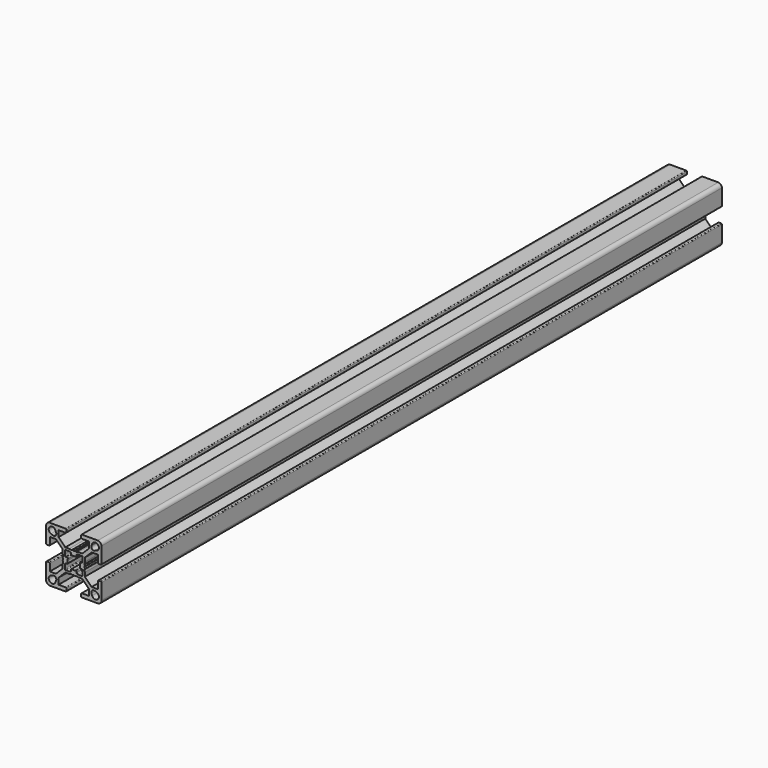
from build123d import *

# Parameters (mm, degrees)
F1_DEPTH = 420


# Not quite as in the source:
# - ends of sketch curves that miss each other by under 0.0002 mm in the source are joined


with BuildPart() as f1:
    # F0 (on Front) → F1 (new body)
    with BuildSketch(Plane.XZ):
        with BuildLine():
            ThreePointArc((21.683673, 22.959406), (21.8008302875, 23.2422487125), (22.083673, 23.359406))
            Line((22.083673, 23.359406), (23.829607, 23.359406))
            ThreePointArc((23.829607, 23.359406), (23.8679454853, 23.3575644616), (23.9059309617, 23.3520568027))
            Line((23.9059309617, 23.3520568027), (24.659993, 23.205482))
            ThreePointArc((24.659993, 23.205482), (24.8923196389, 23.067262524), (24.98367, 22.812831))
            Line((24.98367, 22.812831), (24.98367, 22.196712))
            ThreePointArc((24.98367, 22.196712), (25.1452540389, 21.8755300741), (25.4994591475, 21.8138375123))
            ThreePointArc((25.4994591475, 21.8138375123), (25.9862111121, 21.9228171635), (26.48367, 21.959406))
            Line((26.48367, 21.959406), (26.48367, 24.259406))
            Line((26.48367, 24.259406), (26.080079, 24.492418))
            ThreePointArc((26.080079, 24.492418), (25.830079, 24.559406), (25.5800791291, 24.4924187764))
            Line((25.5800791291, 24.4924187764), (25.264783, 24.310382))
            Line((25.264783, 24.310382), (23.98367, 24.559406))
            Line((23.98367, 24.559406), (21.897875, 24.559406))
            Line((21.897875, 24.559406), (18.23367, 28.223612))
            Line((18.23367, 28.223612), (18.23367, 31.559402))
            Line((18.23367, 31.559402), (22.083673, 31.559402))
            ThreePointArc((22.083673, 31.559402), (22.3665157125, 31.6765592875), (22.483673, 31.959402))
            Line((22.483673, 31.959402), (22.483673, 33.159402))
            ThreePointArc((22.483673, 33.159402), (22.3665157125, 33.4422447125), (22.083673, 33.559402))
            Line((22.083673, 33.559402), (13.483674, 33.559402))
            ThreePointArc((13.483674, 33.559402), (12.0694604376, 32.9736155624), (11.483674, 31.559402))
            Line((11.483674, 31.559402), (11.483674, 22.959403))
            ThreePointArc((11.483674, 22.959403), (11.6008312875, 22.6765602875), (11.883674, 22.559403))
            Line((11.883674, 22.559403), (13.083674, 22.559403))
            ThreePointArc((13.083674, 22.559403), (13.3665167125, 22.6765602875), (13.483674, 22.959403))
            Line((13.483674, 22.959403), (13.483674, 26.809406))
            Line((13.483674, 26.809406), (16.819447, 26.809406))
            Line((16.819447, 26.809406), (20.48367, 23.145184))
            Line((20.48367, 23.145184), (20.48367, 21.059406))
            Line((20.48367, 21.059406), (20.732693, 19.778291))
            Line((20.732693, 19.778291), (20.550657, 19.462994))
            ThreePointArc((20.550657, 19.462994), (20.48367, 19.212994), (20.5506572236, 18.9629941291))
            Line((20.5506572236, 18.9629941291), (20.78367, 18.559405))
            Line((20.78367, 18.559405), (23.08367, 18.559406))
            ThreePointArc((23.08367, 18.559406), (23.1202587453, 19.0568642713), (23.2292374892, 19.543615852))
            ThreePointArc((23.2292374892, 19.543615852), (23.1675451248, 19.897821693), (22.846363, 20.059406))
            Line((22.846363, 20.059406), (22.230245, 20.059406))
            ThreePointArc((22.230245, 20.059406), (21.9758138548, 20.1507560489), (21.8375941973, 20.3830820383))
            Line((21.8375941973, 20.3830820383), (21.691022, 21.137129))
            ThreePointArc((21.691022, 21.137129), (21.6855145384, 21.1751145147), (21.683673, 21.213453))
            Line((21.683673, 21.213453), (21.683673, 22.959406))
        make_face()
        with BuildLine():
            ThreePointArc((14.1338310917, 28.473990252), (13.440167448, 31.6029092165), (16.5690860694, 30.9092440253))
            Line((16.5690860694, 30.9092440253), (16.935818, 29.901655))
            ThreePointArc((16.935818, 29.901655), (16.610197705, 28.4328777176), (15.1414197615, 28.1072573447))
            Line((15.1414197615, 28.1072573447), (14.1338310917, 28.473990252))
        make_face(mode=Mode.SUBTRACT)
        with BuildLine():
            Line((26.48367, 24.259406), (26.48367, 21.959406))
            ThreePointArc((26.48367, 21.959406), (26.9811284145, 21.9228172335), (27.4678801291, 21.813838427))
            ThreePointArc((27.4678801291, 21.813838427), (27.8220855768, 21.8755297889), (27.98367, 22.196712))
            Line((27.98367, 22.196712), (27.98367, 22.812831))
            ThreePointArc((27.98367, 22.812831), (28.0750200489, 23.0672621452), (28.3073460383, 23.2054818027))
            Line((28.3073460383, 23.2054818027), (29.061393, 23.352053))
            ThreePointArc((29.061393, 23.352053), (29.0993785147, 23.3575614616), (29.137717, 23.359403))
            Line((29.137717, 23.359403), (30.88367, 23.359403))
            ThreePointArc((30.88367, 23.359403), (31.1665127125, 23.2422457125), (31.28367, 22.959403))
            Line((31.28367, 22.959403), (31.28367, 21.213468))
            ThreePointArc((31.28367, 21.213468), (31.2818285086, 21.1751300032), (31.27632099, 21.1371450019))
            Line((31.27632099, 21.1371450019), (31.129746, 20.383082))
            ThreePointArc((31.129746, 20.383082), (30.9915261452, 20.1507560489), (30.737095, 20.059406))
            Line((30.737095, 20.059406), (30.120976, 20.059406))
            ThreePointArc((30.120976, 20.059406), (29.7997937889, 19.8978215768), (29.7381017894, 19.5436159363))
            ThreePointArc((29.7381017894, 19.5436159363), (29.8470812335, 19.0568644145), (29.88367, 18.559406))
            Line((29.88367, 18.559406), (32.18367, 18.559406))
            Line((32.18367, 18.559406), (32.416682, 18.962996))
            ThreePointArc((32.416682, 18.962996), (32.48367, 19.212996), (32.4166825264, 19.4629963039))
            Line((32.4166825264, 19.4629963039), (32.234646, 19.778292))
            Line((32.234646, 19.778292), (32.48367, 21.059406))
            Line((32.48367, 21.059406), (32.48367, 23.1452))
            Line((32.48367, 23.1452), (36.147876, 26.809406))
            Line((36.147876, 26.809406), (39.483666, 26.809406))
            Line((39.483666, 26.809406), (39.483666, 22.959403))
            ThreePointArc((39.483666, 22.959403), (39.6008232875, 22.6765602875), (39.883666, 22.559403))
            Line((39.883666, 22.559403), (41.083666, 22.559403))
            ThreePointArc((41.083666, 22.559403), (41.3665087125, 22.6765602875), (41.483666, 22.959403))
            Line((41.483666, 22.959403), (41.483666, 31.559402))
            ThreePointArc((41.483666, 31.559402), (40.8978795624, 32.9736155624), (39.483666, 33.559402))
            Line((39.483666, 33.559402), (30.883667, 33.559402))
            ThreePointArc((30.883667, 33.559402), (30.6008242875, 33.4422447125), (30.483667, 33.159402))
            Line((30.483667, 33.159402), (30.483667, 31.959402))
            ThreePointArc((30.483667, 31.959402), (30.6008242875, 31.6765592875), (30.883667, 31.559402))
            Line((30.883667, 31.559402), (34.73367, 31.559402))
            Line((34.73367, 31.559402), (34.73367, 28.223628))
            Line((34.73367, 28.223628), (31.069448, 24.559406))
            Line((31.069448, 24.559406), (28.98367, 24.559406))
            Line((28.98367, 24.559406), (27.702555, 24.310382))
            Line((27.702555, 24.310382), (27.387259, 24.492418))
            ThreePointArc((27.387259, 24.492418), (27.137259, 24.559406), (26.8872591291, 24.4924187764))
            Line((26.8872591291, 24.4924187764), (26.48367, 24.259406))
        make_face()
        with BuildLine():
            ThreePointArc((36.3982539306, 30.9092440253), (39.5271728843, 31.6029088843), (38.8335080253, 28.4739899306))
            Line((38.8335080253, 28.4739899306), (37.825919, 28.107257))
            ThreePointArc((37.825919, 28.107257), (36.3571411741, 28.4328778386), (36.0315216661, 29.9016561215))
            Line((36.0315216661, 29.9016561215), (36.3982539306, 30.9092440253))
        make_face(mode=Mode.SUBTRACT)
        with BuildLine():
            ThreePointArc((23.2292377663, 17.5751952317), (23.1202588153, 18.0619472552), (23.08367, 18.559406))
            Line((23.08367, 18.559406), (20.78367, 18.559406))
            Line((20.78367, 18.559406), (20.550657, 18.155815))
            ThreePointArc((20.550657, 18.155815), (20.48367, 17.905815), (20.5506572236, 17.6558151291))
            Line((20.5506572236, 17.6558151291), (20.732693, 17.340519))
            Line((20.732693, 17.340519), (20.48367, 16.059406))
            Line((20.48367, 16.059406), (20.48367, 13.973611))
            Line((20.48367, 13.973611), (16.819464, 10.309406))
            Line((16.819464, 10.309406), (13.483674, 10.309406))
            Line((13.483674, 10.309406), (13.483674, 14.159409))
            ThreePointArc((13.483674, 14.159409), (13.3665167125, 14.4422517125), (13.083674, 14.559409))
            Line((13.083674, 14.559409), (11.883674, 14.559409))
            ThreePointArc((11.883674, 14.559409), (11.6008312875, 14.4422517125), (11.483674, 14.159409))
            Line((11.483674, 14.159409), (11.483674, 5.55941))
            ThreePointArc((11.483674, 5.55941), (12.0694604376, 4.1451964376), (13.483674, 3.55941))
            Line((13.483674, 3.55941), (22.083673, 3.55941))
            ThreePointArc((22.083673, 3.55941), (22.3665157125, 3.6765672875), (22.483673, 3.95941))
            Line((22.483673, 3.95941), (22.483673, 5.15941))
            ThreePointArc((22.483673, 5.15941), (22.3665157125, 5.4422527125), (22.083673, 5.55941))
            Line((22.083673, 5.55941), (18.23367, 5.55941))
            Line((18.23367, 5.55941), (18.23367, 8.895183))
            Line((18.23367, 8.895183), (21.897891, 12.559406))
            Line((21.897891, 12.559406), (23.98367, 12.559406))
            Line((23.98367, 12.559406), (25.264785, 12.808429))
            Line((25.264785, 12.808429), (25.580081, 12.626393))
            ThreePointArc((25.580081, 12.626393), (25.830081, 12.559406), (26.0800808709, 12.6263932236))
            Line((26.0800808709, 12.6263932236), (26.483671, 12.859406))
            Line((26.483671, 12.859406), (26.48367, 15.159406))
            ThreePointArc((26.48367, 15.159406), (25.9862111121, 15.1959948365), (25.4994589547, 15.3049738501))
            ThreePointArc((25.4994589547, 15.3049738501), (25.1452540389, 15.2432809259), (24.98367, 14.922099))
            Line((24.98367, 14.922099), (24.98367, 14.305981))
            ThreePointArc((24.98367, 14.305981), (24.8923196389, 14.051549476), (24.6599929981, 13.91333001))
            Line((24.6599929981, 13.91333001), (23.905946, 13.766758))
            ThreePointArc((23.905946, 13.766758), (23.8679609968, 13.7612504914), (23.829623, 13.759409))
            Line((23.829623, 13.759409), (22.08367, 13.759409))
            ThreePointArc((22.08367, 13.759409), (21.8008272875, 13.8765662875), (21.68367, 14.159409))
            Line((21.68367, 14.159409), (21.68367, 15.905343))
            ThreePointArc((21.68367, 15.905343), (21.6855115384, 15.9436814853), (21.6910191973, 15.9816669617))
            Line((21.6910191973, 15.9816669617), (21.837594, 16.735729))
            ThreePointArc((21.837594, 16.735729), (21.975813476, 16.9680556389), (22.230245, 17.059406))
            Line((22.230245, 17.059406), (22.846363, 17.059406))
            ThreePointArc((22.846363, 17.059406), (23.1675448396, 17.2209899227), (23.2292377663, 17.5751952317))
        make_face()
        with BuildLine():
            ThreePointArc((16.5690860694, 6.2095679747), (13.440167448, 5.5159027835), (14.1338310917, 8.644821748))
            Line((14.1338310917, 8.644821748), (15.14142, 9.011554))
            ThreePointArc((15.14142, 9.011554), (16.6101974937, 8.6859334937), (16.9358177723, 7.2171560829))
            Line((16.9358177723, 7.2171560829), (16.5690860694, 6.2095679747))
        make_face(mode=Mode.SUBTRACT)
        with BuildLine():
            ThreePointArc((27.4678801291, 15.304973573), (26.9811284145, 15.1959947665), (26.48367, 15.159406))
            Line((26.48367, 15.159406), (26.48367, 12.859406))
            Line((26.48367, 12.859406), (26.887261, 12.626393))
            ThreePointArc((26.887261, 12.626393), (27.137261, 12.559406), (27.3872608709, 12.6263932236))
            Line((27.3872608709, 12.6263932236), (27.702556, 12.808429))
            Line((27.702556, 12.808429), (28.98367, 12.559406))
            Line((28.98367, 12.559406), (31.069464, 12.559406))
            Line((31.069464, 12.559406), (34.73367, 8.8952))
            Line((34.73367, 8.8952), (34.73367, 5.55941))
            Line((34.73367, 5.55941), (30.883667, 5.55941))
            ThreePointArc((30.883667, 5.55941), (30.6008242875, 5.4422527125), (30.483667, 5.15941))
            Line((30.483667, 5.15941), (30.483667, 3.95941))
            ThreePointArc((30.483667, 3.95941), (30.6008242875, 3.6765672875), (30.883667, 3.55941))
            Line((30.883667, 3.55941), (39.483666, 3.55941))
            ThreePointArc((39.483666, 3.55941), (40.8978795624, 4.1451964376), (41.483666, 5.55941))
            Line((41.483666, 5.55941), (41.483666, 14.159409))
            ThreePointArc((41.483666, 14.159409), (41.3665087125, 14.4422517125), (41.083666, 14.559409))
            Line((41.083666, 14.559409), (39.883666, 14.559409))
            ThreePointArc((39.883666, 14.559409), (39.6008232875, 14.4422517125), (39.483666, 14.159409))
            Line((39.483666, 14.159409), (39.483666, 10.309406))
            Line((39.483666, 10.309406), (36.147892, 10.309406))
            Line((36.147892, 10.309406), (32.48367, 13.973627))
            Line((32.48367, 13.973627), (32.48367, 16.059406))
            Line((32.48367, 16.059406), (32.234646, 17.340521))
            Line((32.234646, 17.340521), (32.416682, 17.655817))
            ThreePointArc((32.416682, 17.655817), (32.48367, 17.905817), (32.4166825264, 18.1558173039))
            Line((32.4166825264, 18.1558173039), (32.18367, 18.559407))
            Line((32.18367, 18.559407), (29.88367, 18.559406))
            ThreePointArc((29.88367, 18.559406), (29.8470811635, 18.0619471121), (29.7381021499, 17.5751949547))
            ThreePointArc((29.7381021499, 17.5751949547), (29.7997940741, 17.2209900389), (30.120976, 17.059406))
            Line((30.120976, 17.059406), (30.737095, 17.059406))
            ThreePointArc((30.737095, 17.059406), (30.991526524, 16.9680556389), (31.12974599, 16.7357289981))
            Line((31.12974599, 16.7357289981), (31.276318, 15.981682))
            ThreePointArc((31.276318, 15.981682), (31.2818255086, 15.9436969968), (31.283667, 15.905359))
            Line((31.283667, 15.905359), (31.283667, 14.159406))
            ThreePointArc((31.283667, 14.159406), (31.1665097125, 13.8765632875), (30.883667, 13.759406))
            Line((30.883667, 13.759406), (29.137732, 13.759406))
            ThreePointArc((29.137732, 13.759406), (29.0993940032, 13.7612474914), (29.0614090019, 13.76675501))
            Line((29.0614090019, 13.76675501), (28.307346, 13.91333))
            ThreePointArc((28.307346, 13.91333), (28.0750200489, 14.0515498548), (27.98367, 14.305981))
            Line((27.98367, 14.305981), (27.98367, 14.922099))
            ThreePointArc((27.98367, 14.922099), (27.8220855768, 15.2432812111), (27.4678801291, 15.304973573))
        make_face()
        with BuildLine():
            ThreePointArc((38.8335080253, 8.6448220694), (39.5271728843, 5.5159031157), (36.3982539306, 6.2095679747))
            Line((36.3982539306, 6.2095679747), (36.031521, 7.217156))
            ThreePointArc((36.031521, 7.217156), (36.3571413854, 8.6859333727), (37.8259189171, 9.0115537723))
            Line((37.8259189171, 9.0115537723), (38.8335080253, 8.6448220694))
        make_face(mode=Mode.SUBTRACT)
    extrude(amount=F1_DEPTH)


solid = f1.part
